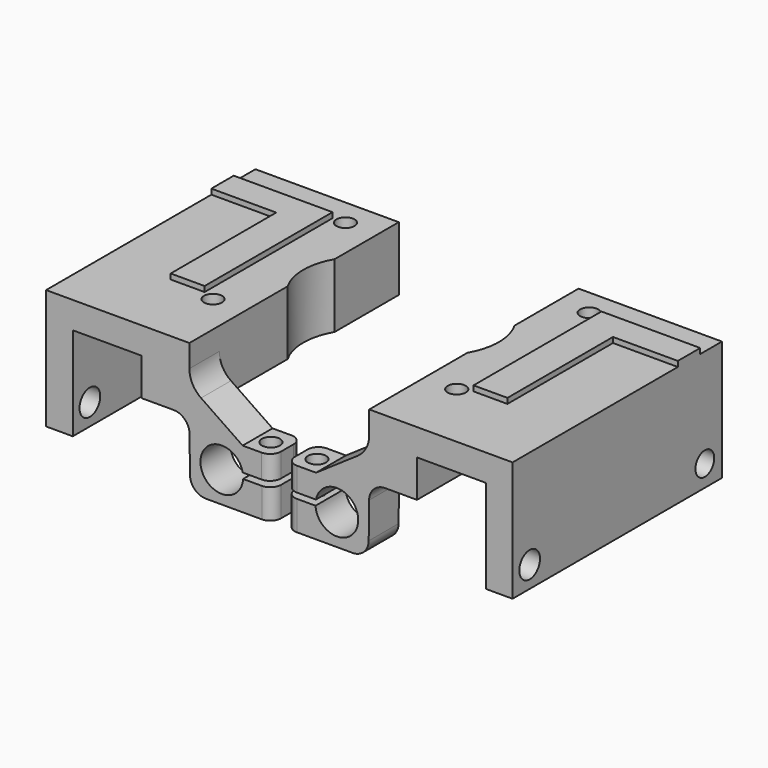
from build123d import *

# Parameters (mm, degrees)
F1_DEPTH      = 7
F2_DEPTH      = 42
F3_R          = 1.7
F3_R_2        = 11
F4_DEPTH      = 12.001
F5_R          = 4
F6_DEPTH      = 10
F7_DEPTH      = 12.001
F8_R          = 1.4
F9_DEPTH      = 10.9920075553
F8_R_2        = 1.7
F10_DEPTH     = 4.4348209087
F11_R         = 5
F12_R         = 3
F13_R         = 3
F14_R         = 2
F15_R         = 2.2
F15_R_2       = 2.4255023423
F16_DEPTH     = 6
F17_TEXT_SIZE = 41.9437823343
F18_DEPTH     = 1


# Not quite as in the source:
# - a feature names something its author has since deleted; it is built from what else it names
# - Text() gives the source's letters only with a copy of the font that has no kerning and outlines rounded to 1/6400 em; it was checked with that copy


with BuildPart() as f1:
    # F0 (on Front) → F1 (new body)
    with BuildSketch(Plane.XZ):
        Polygon((-18.6721007523, 29.8099789735), (-18.6721007523, 7.3259699669), (-13.6721007523, 7.3259699669), (-13.6721007523, 24.8099789735), (-0.7721007523, 24.8099789735), (-0.7721007523, 17.8099789735), (8.1637966118, 17.8099789735), (8.1637966118, 22.9406704692), (8.1637966118, 29.8099789735), align=None)
        Polygon((18.1301751077, 16.1394868046), (8.1637966118, 22.9406704692), (8.1637966118, 17.8099789735), (8.2940201178, 5.1484792493), (23.7186601057, 5.1484792493), (23.7186601057, 10.6682249423), (16.3860510706, 10.6682249423), (16.3860510706, 11.7046658959), (23.6896428882, 11.7046658959), (23.6896428882, 16.1394868046), align=None)
    extrude(amount=F1_DEPTH)

    # F0 (on Front) → F2 (join)
    with BuildSketch(Plane.XZ):
        Polygon((-18.6721007523, 29.8099789735), (-18.6721007523, 7.3259699669), (-13.6721007523, 7.3259699669), (-13.6721007523, 24.8099789735), (-0.7721007523, 24.8099789735), (-0.7721007523, 17.8099789735), (8.1637966118, 17.8099789735), (8.1637966118, 22.9406704692), (8.1637966118, 29.8099789735), align=None)
    extrude(amount=-F2_DEPTH)

    # F3 (on face) → F4 (cut, through all)
    with BuildSketch(Plane(origin=(0, 0, 17.8099789735), x_dir=(1, 0, 0), z_dir=(0, 0, -1))):
        with Locations((2.1850741468, -6)):
            Circle(F3_R)
        with Locations((2.1850741468, -37)):
            Circle(F3_R)
        with Locations((17.6850741468, -21.5)):
            Circle(F3_R_2)
    extrude(amount=-F4_DEPTH, mode=Mode.SUBTRACT)

    # F5 (on face) → F6 (cut)
    with BuildSketch(Plane.XZ.offset(7)):
        with Locations((14.2278992477, 10.8989789735)):
            Circle(F5_R)
    extrude(amount=-F6_DEPTH, mode=Mode.SUBTRACT)

    # F3 (on face) → F7 (cut, through all)
    with BuildSketch(Plane(origin=(0, 0, 17.8099789735), x_dir=(1, 0, 0), z_dir=(0, 0, -1))):
        with Locations((2.1850741468, -6)):
            Circle(F3_R)
        with Locations((2.1850741468, -37)):
            Circle(F3_R)
        with Locations((17.6850741468, -21.5)):
            Circle(F3_R_2)
    extrude(amount=-F7_DEPTH, mode=Mode.SUBTRACT)

    # F8 (on face) → F9 (cut, through all)
    with BuildSketch(Plane.XY.offset(16.1394868046)):
        with Locations((20.6896428882, -3.5767070949)):
            Circle(F8_R)
    extrude(amount=-F9_DEPTH, mode=Mode.SUBTRACT)

    # F8 (on face) → F10 (cut, through all)
    with BuildSketch(Plane.XY.offset(16.1394868046)):
        with Locations((20.6896428882, -3.5767070949)):
            Circle(F8_R_2)
        with Locations((20.6896428882, -3.5767070949)):
            Circle(F8_R, mode=Mode.SUBTRACT)
    extrude(amount=-F10_DEPTH, mode=Mode.SUBTRACT)

    # F11
    f11_edges = [f1.edges().sort_by_distance(p)[0] for p in [
        (8.163797, -3.5, 22.94067),
    ]]
    fillet(f11_edges, radius=F11_R)

    # F12
    f12_edges = [f1.edges().sort_by_distance(p)[0] for p in [
        (8.163797, -3.5, 17.809979),
    ]]
    fillet(f12_edges, radius=F12_R)

    # F13
    f13_edges = [f1.edges().sort_by_distance(p)[0] for p in [
        (8.29402, -3.5, 5.148479),
    ]]
    fillet(f13_edges, radius=F13_R)

    # F14
    f14_edges = [f1.edges().sort_by_distance(p)[0] for p in [
        (23.689643, -7, 13.922076),
        (23.71866, -7, 7.908352),
        (23.689643, 0, 13.922076),
        (23.71866, 0, 7.908352),
    ]]
    fillet(f14_edges, radius=F14_R)

    # F15 (on face) → F16 (cut)
    with BuildSketch(Plane(origin=(-18.6721007523, 0, 0), x_dir=(0, -1, 0), z_dir=(-1, 0, 0))):
        with Locations((-38, 11.3259699669)):
            Circle(F15_R)
        with Locations((3, 11.3259699669)):
            Circle(F15_R_2)
    extrude(amount=-F16_DEPTH, mode=Mode.SUBTRACT)

    # F17 (on face) → F18 (join)
    with BuildSketch(Plane.XY.offset(29.8099789735)):
        with Locations(Location((3.5908724648, 36.9253193088), (0, 0, 180))):
            Text('L', F17_TEXT_SIZE, font='Open Sans', font_style=FontStyle.BOLD, text_align=(TextAlign.LEFT, TextAlign.BOTTOM))
    extrude(amount=F18_DEPTH)


with BuildPart() as f19_1:
    # F19: instance of F1
    add(f1.part.mirror(Plane.YZ))


with BuildPart() as f19_1_1:
    # F20: moved
    add(f19_1.part.moved(Location((50, 0, 0))))


solid = Compound([f1.part, f19_1_1.part])
